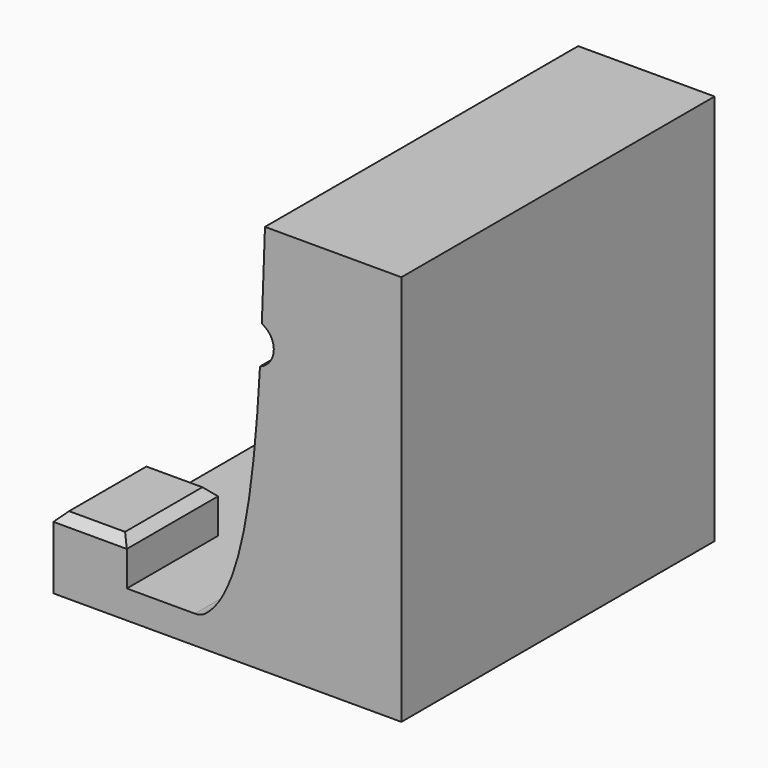
from build123d import *

# Parameters (mm, degrees)
F7_DEPTH = 114.3
F0_W     = 21.425565113
F0_H     = 33.2948663116
F8_DEPTH = 12.7
F0_H_2   = 38.15253824
F9_DEPTH = 12.7
F10_SIZE = 2.54
F1_SIZE  = 2.54
F11_SIZE = 2.54
F2_SIZE  = 2.54
F12_SIZE = 2.54
F3_SIZE  = 2.54
F4_SIZE  = 2.54
F13_R    = 5.08


# Not quite as in the source:
# - a feature of the source that left no trace in its solid (it failed there, or was rolled back) is left out


with BuildPart() as f7:
    # F6 (on Front) → F7 (new body)
    with BuildSketch(Plane.XZ):
        with BuildLine():
            Line((28.0298027718, 88.895993849), (-11.7995445112, 88.895993849))
            add(Edge.make_bspline(
                [(-12.7191172273, 63.6731384112), (-12.3630729131, 71.9399928392), (-12.0813087773, 80.417993931), (-11.7995445112, 88.895993849)],
                knots=[0.894750445, 0.894750445, 0.894750445, 0.894750445, 1, 1, 1, 1], degree=3))
            ThreePointArc((-12.7191172273, 63.6731384112), (-9.233937312, 57.9257119158), (-13.2581382148, 52.5419216657))
            add(Edge.make_bspline(
                [(-30.7190670022, -17.1741323863), (-19.0091812538, -10.6770336575), (-15.1403430342, 18.1088676273), (-13.2581382148, 52.5419216657)],
                knots=[0.3956141416, 0.3956141416, 0.3956141416, 0.3956141416, 0.846870688, 0.846870688, 0.846870688, 0.846870688], degree=3))
            add(Edge.make_bspline(
                [(-44.7375965866, -17.1741323863), (-39.4125863388, -19.0279691828), (-34.6287794117, -19.3433924519), (-30.7190670022, -17.1741323863)],
                knots=[0.2449479988, 0.2449479988, 0.2449479988, 0.2449479988, 0.3956141416, 0.3956141416, 0.3956141416, 0.3956141416], degree=3))
            Line((-44.7375965866, -17.1741323863), (-49.7875006466, -17.1741323863))
            Line((-49.7875006466, -17.1741323863), (-73.5701972282, -17.1741323863))
            Line((-73.5701972282, -17.1741323863), (-73.5701972282, -25.404006151))
            Line((-73.5701972282, -25.404006151), (28.0298027718, -25.404006151))
            Line((28.0298027718, -25.404006151), (28.0298027718, 88.895993849))
        make_face()
        with BuildLine():
            add(Edge.make_bspline(
                [(-44.7375965866, -17.1741323863), (-39.4125863388, -19.0279691828), (-34.6287794117, -19.3433924519), (-30.7190670022, -17.1741323863)],
                knots=[0.2449479988, 0.2449479988, 0.2449479988, 0.2449479988, 0.3956141416, 0.3956141416, 0.3956141416, 0.3956141416], degree=3))
            Line((-30.7190670022, -17.1741323863), (-44.7375965866, -17.1741323863))
        make_face()
    extrude(amount=F7_DEPTH)

    # F0 (on face) → F8 (join)
    with BuildSketch(Plane.XY.offset(-17.1741323863)):
        with Locations((-62.8574146717, -97.6525668442)):
            Rectangle(F0_W, F0_H)
    extrude(amount=F8_DEPTH)

    # F0 (on face) → F9 (join)
    with BuildSketch(Plane.XY.offset(-17.1741323863)):
        with Locations((-62.8574146717, -19.07626912)):
            Rectangle(F0_W, F0_H_2)
    extrude(amount=F9_DEPTH)

    # F10
    f10_edges = [f7.edges().sort_by_distance(p)[0] for p in [
        (-62.857415, 0, -4.474132),
    ]]
    chamfer(f10_edges, length=F10_SIZE)

    # F1
    f1_edges = [f7.edges().sort_by_distance(p)[0] for p in [
        (-52.144632, -20.346269, -4.474132),
        (-52.144632, -97.652567, -4.474132),
    ]]
    chamfer(f1_edges, length=F1_SIZE)

    # F11
    f11_edges = [f7.edges().sort_by_distance(p)[0] for p in [
        (-73.570197, -20.346269, -4.474132),
    ]]
    chamfer(f11_edges, length=F11_SIZE)

    # F2
    f2_edges = [f7.edges().sort_by_distance(p)[0] for p in [
        (-62.857415, -38.152538, -4.474132),
    ]]
    chamfer(f2_edges, length=F2_SIZE)

    # F12
    f12_edges = [f7.edges().sort_by_distance(p)[0] for p in [
        (-64.127415, -114.3, -4.474132),
    ]]
    chamfer(f12_edges, length=F12_SIZE)

    # F3
    f3_edges = [f7.edges().sort_by_distance(p)[0] for p in [
        (-73.570197, -96.382567, -4.474132),
    ]]
    chamfer(f3_edges, length=F3_SIZE)

    # F4
    f4_edges = [f7.edges().sort_by_distance(p)[0] for p in [
        (-62.857415, -81.005134, -4.474132),
    ]]
    chamfer(f4_edges, length=F4_SIZE)

    # F13
    f13_edges = [f7.edges().sort_by_distance(p)[0] for p in [
        (-30.719067, -57.15, -17.174132),
    ]]
    fillet(f13_edges, radius=F13_R)


solid = f7.part
